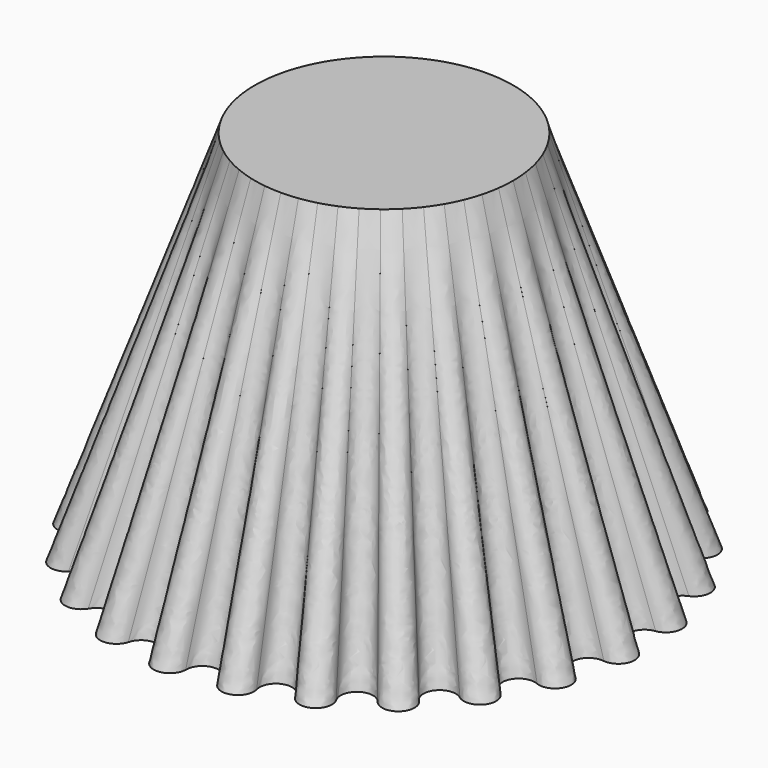
from build123d import *

# Parameters (mm, degrees)
F2_R = 317.5


with BuildPart() as f4:
    # F0 (on Top) → F4 section 0
    with BuildSketch(Plane.XY):
        with BuildLine():
            ThreePointArc((-588.8283837058, 157.7760898945), (-558.7620975694, 111.1446916296), (-604.3847874935, 79.5687667773))
            ThreePointArc((-604.3847874935, 79.5687667773), (-648.100495463, 42.4787507249), (-609.6, 0))
            ThreePointArc((-609.6, 0), (-568.4891037495, -37.2607444325), (-604.3847874935, -79.5687667773))
            ThreePointArc((-604.3847874935, -79.5687667773), (-637.0113162982, -126.7094289725), (-588.8283837058, -157.7760898945))
            ThreePointArc((-588.8283837058, -157.7760898945), (-539.4745169818, -183.1269223377), (-563.1969630189, -233.2838203698))
            ThreePointArc((-563.1969630189, -233.2838203698), (-582.5108686387, -287.2625704827), (-527.929086147, -304.8))
            ThreePointArc((-527.929086147, -304.8), (-473.6956334055, -316.5133031172), (-483.6281962415, -371.1009671237))
            ThreePointArc((-483.6281962415, -371.1009671237), (-488.3132679262, -428.2392425383), (-431.0522938113, -431.0522938113))
            ThreePointArc((-431.0522938113, -431.0522938113), (-375.6351752317, -428.3298253522), (-371.1009671237, -483.6281962415))
            ThreePointArc((-371.1009671237, -483.6281962415), (-360.8379249803, -540.0321179138), (-304.8, -527.929086147))
            ThreePointArc((-304.8, -527.929086147), (-251.9758006323, -510.956377838), (-233.2838203698, -563.1969630189))
            ThreePointArc((-233.2838203698, -563.1969630189), (-208.7720737599, -615.0226968987), (-157.7760898945, -588.8283837058))
            ThreePointArc((-157.7760898945, -588.8283837058), (-111.1446916296, -558.7620975694), (-79.5687667773, -604.3847874935))
            ThreePointArc((-79.5687667773, -604.3847874935), (-42.4787507249, -648.100495463), (0, -609.6))
            ThreePointArc((0, -609.6), (37.2607444325, -568.4891037495), (79.5687667773, -604.3847874935))
            ThreePointArc((79.5687667773, -604.3847874935), (126.7094289725, -637.0113162982), (157.7760898945, -588.8283837058))
            ThreePointArc((157.7760898945, -588.8283837058), (183.1269223377, -539.4745169818), (233.2838203698, -563.1969630189))
            ThreePointArc((233.2838203698, -563.1969630189), (287.2625704827, -582.5108686387), (304.8, -527.929086147))
            ThreePointArc((304.8, -527.929086147), (316.5133031172, -473.6956334055), (371.1009671237, -483.6281962415))
            ThreePointArc((371.1009671237, -483.6281962415), (428.2392425383, -488.3132679262), (431.0522938113, -431.0522938113))
            ThreePointArc((431.0522938113, -431.0522938113), (428.3298253522, -375.6351752317), (483.6281962415, -371.1009671237))
            ThreePointArc((483.6281962415, -371.1009671237), (540.0321179138, -360.8379249803), (527.929086147, -304.8))
            ThreePointArc((527.929086147, -304.8), (510.956377838, -251.9758006323), (563.1969630189, -233.2838203698))
            ThreePointArc((563.1969630189, -233.2838203698), (615.0226968987, -208.7720737599), (588.8283837058, -157.7760898945))
            ThreePointArc((588.8283837058, -157.7760898945), (558.7620975694, -111.1446916296), (604.3847874935, -79.5687667773))
            ThreePointArc((604.3847874935, -79.5687667773), (648.100495463, -42.4787507249), (609.6, 0))
            ThreePointArc((609.6, 0), (568.4891037495, 37.2607444325), (604.3847874935, 79.5687667773))
            ThreePointArc((604.3847874935, 79.5687667773), (637.0113162982, 126.7094289725), (588.8283837058, 157.7760898945))
            ThreePointArc((588.8283837058, 157.7760898945), (539.4745169818, 183.1269223377), (563.1969630189, 233.2838203698))
            ThreePointArc((563.1969630189, 233.2838203698), (582.5108686387, 287.2625704827), (527.929086147, 304.8))
            ThreePointArc((527.929086147, 304.8), (473.6956334055, 316.5133031172), (483.6281962415, 371.1009671237))
            ThreePointArc((483.6281962415, 371.1009671237), (488.3132679262, 428.2392425383), (431.0522938113, 431.0522938113))
            ThreePointArc((431.0522938113, 431.0522938113), (375.6351752317, 428.3298253522), (371.1009671237, 483.6281962415))
            ThreePointArc((371.1009671237, 483.6281962415), (360.8379249803, 540.0321179138), (304.8, 527.929086147))
            ThreePointArc((304.8, 527.929086147), (251.9758006323, 510.956377838), (233.2838203698, 563.1969630189))
            ThreePointArc((233.2838203698, 563.1969630189), (208.7720737599, 615.0226968987), (157.7760898945, 588.8283837058))
            ThreePointArc((157.7760898945, 588.8283837058), (111.1446916296, 558.7620975694), (79.5687667773, 604.3847874935))
            ThreePointArc((79.5687667773, 604.3847874935), (42.4787507249, 648.100495463), (0, 609.6))
            ThreePointArc((0, 609.6), (-37.2607444325, 568.4891037495), (-79.5687667773, 604.3847874935))
            ThreePointArc((-79.5687667773, 604.3847874935), (-126.7094289725, 637.0113162982), (-157.7760898945, 588.8283837058))
            ThreePointArc((-157.7760898945, 588.8283837058), (-183.1269223377, 539.4745169818), (-233.2838203698, 563.1969630189))
            ThreePointArc((-233.2838203698, 563.1969630189), (-287.2625704827, 582.5108686387), (-304.8, 527.929086147))
            ThreePointArc((-304.8, 527.929086147), (-316.5133031172, 473.6956334055), (-371.1009671237, 483.6281962415))
            ThreePointArc((-371.1009671237, 483.6281962415), (-428.2392425383, 488.3132679262), (-431.0522938113, 431.0522938113))
            ThreePointArc((-431.0522938113, 431.0522938113), (-428.3298253522, 375.6351752317), (-483.6281962415, 371.1009671237))
            ThreePointArc((-483.6281962415, 371.1009671237), (-540.0321179138, 360.8379249803), (-527.929086147, 304.8))
            ThreePointArc((-527.929086147, 304.8), (-510.956377838, 251.9758006323), (-563.1969630189, 233.2838203698))
            ThreePointArc((-563.1969630189, 233.2838203698), (-615.0226968987, 208.7720737599), (-588.8283837058, 157.7760898945))
        make_face()
    # F2 (on offset) → F4 section 1
    with BuildSketch(Plane.XY.offset(914.4)):
        Circle(F2_R)
    loft()


solid = f4.part
